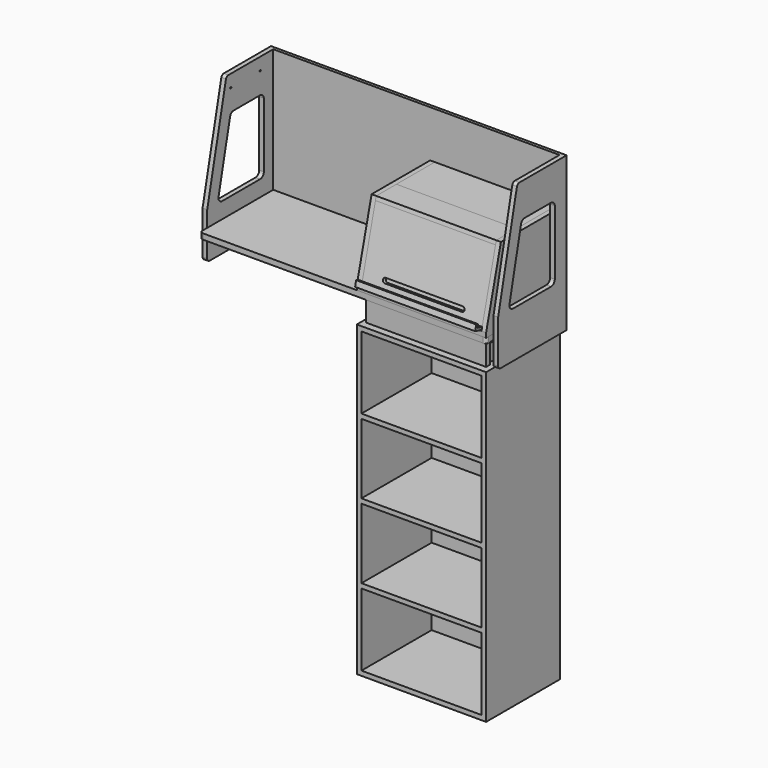
from build123d import *

# Parameters (mm, degrees)
F0_W           = 15
F0_H           = 500
F1_DEPTH       = 8
F2_DEPTH       = 270
F3_SIZE2       = 78
F3_SIZE        = 350
F3_2_SIZE2     = 78
F3_2_SIZE      = 350
F4_W           = 270
F4_H           = 18
F4_W_2         = 30
F5_DEPTH       = 930
F6_R           = 10
F6_2_R         = 10
F7_W           = 15
F7_H           = 235
F7_H_2         = 15
F7_W_2         = 390
F8_DEPTH       = 300
F9_DEPTH       = 8
F10_SIZE2      = 60
F10_SIZE       = 235
F11_W          = 158
F11_H          = 12
F12_DEPTH      = 390
F13_W          = 250
F13_H          = 15
F14_DEPTH      = 25
F15_DEPTH      = 390
F18_DEPTH      = 15
F19_W          = 348
F19_H          = 8
F20_DEPTH      = 285
F19_W_2        = 8
F19_H_2        = 65
F21_DEPTH      = 285
F22_D          = 5
F22_DEPTH      = 12
F22_TIP        = 1.5021515476
F23_DEPTH      = 25
F23_DEPTH_BACK = 945
F24_R          = 15
F26_DEPTH      = 25
F11_W_2        = 150
F11_H_2        = 8
F28_DEPTH      = 390
F27_W          = 152
F27_H          = 8
F29_DEPTH      = 84
F31_DEPTH      = 2
F32_W          = 420
F32_H          = 300
F33_DEPTH      = 1000
F34_T          = -15
F35_W          = 285
F35_H          = 15
F36_DEPTH      = 390


# Not quite as in the source:
# - a feature names something its author has since deleted; it is built from what else it names


with BuildPart() as f1:
    # F0 (on Front) → F1 (new body)
    with BuildSketch(Plane.XZ):
        with Locations((-952.5, 250)):
            Rectangle(F0_W, F0_H)
        with BuildLine():
            Line((-465, 0), (-15, 0))
            Line((-15, 0), (-15, 500))
            Line((-15, 500), (-945, 500))
            Line((-945, 500), (-945, 0))
            Line((-945, 0), (-495, 0))
            ThreePointArc((-495, 0), (-480, 15), (-465, 0))
        make_face()
        with Locations((-7.5, 250)):
            Rectangle(F0_W, F0_H)
    extrude(amount=-F1_DEPTH)

    # F0 (on Front) → F2 (join)
    with BuildSketch(Plane.XZ):
        with Locations((-952.5, 250)):
            Rectangle(F0_W, F0_H)
        with Locations((-7.5, 250)):
            Rectangle(F0_W, F0_H)
    extrude(amount=F2_DEPTH)

    # F3
    f3_edges = [f1.edges().sort_by_distance(p)[0] for p in [
        (-952.5, -270, 500),
    ]]
    f3_side = f1.faces().sort_by_distance((-952.5, -270, 250))[0]
    chamfer(f3_edges, length=F3_SIZE, length2=F3_SIZE2, reference=f3_side)

    # F3#2
    f3_2_edges = [f1.edges().sort_by_distance(p)[0] for p in [
        (-7.5, -270, 500),
    ]]
    f3_2_side = f1.faces().sort_by_distance((-7.5, -270, 250))[0]
    chamfer(f3_2_edges, length=F3_2_SIZE, length2=F3_2_SIZE2, reference=f3_2_side)

    # F6
    f6_edges = [f1.edges().sort_by_distance(p)[0] for p in [
        (-952.5, -192, 500),
        (-7.5, -192, 500),
        (-7.5, -270, 0),
        (-952.5, -270, 0),
    ]]
    fillet(f6_edges, radius=F6_R)

    # F22 (one way)
    with BuildSketch(Plane.YZ.offset(-945)):
        with Locations((-174.4660586119, 460), (-54.8418462276, 460), (-174.4660586119, 80), (-54.8418462276, 80)):
            Circle(F22_D / 2)
    extrude(amount=-F22_DEPTH, mode=Mode.SUBTRACT)
    with Locations(Plane.YZ.offset(-945)):
        with Locations((-174.4660586119, 460), (-54.8418462276, 460), (-174.4660586119, 80), (-54.8418462276, 80)):
            with Locations((0, 0, -(F22_DEPTH + F22_TIP / 2))):  # 118° drill point
                Cone(0, F22_D / 2, F22_TIP, mode=Mode.SUBTRACT)

    # F4 (on face) → F23 (cut, two sides)
    with BuildSketch(Plane.YZ.offset(-945)) as f23_sk:
        Polygon((-40, 390), (-174.4660586119, 390), (-227.9517728976, 150), (-40, 150), align=None)
    extrude(amount=-F23_DEPTH, mode=Mode.SUBTRACT)
    extrude(f23_sk.sketch, amount=F23_DEPTH_BACK, mode=Mode.SUBTRACT)

    # F24
    f24_edges = [f1.edges().sort_by_distance(p)[0] for p in [
        (-952.5, -40, 150),
        (-952.5, -227.951773, 150),
        (-952.5, -40, 390),
        (-7.5, -227.951773, 150),
        (-7.5, -40, 150),
        (-7.5, -40, 390),
        (-7.5, -174.466059, 390),
        (-952.5, -174.466059, 390),
    ]]
    fillet(f24_edges, radius=F24_R)


with BuildPart() as f5:
    # F4 (on face) → F5 (new body, through all)
    with BuildSketch(Plane.YZ.offset(-945)):
        with Locations((-135, 89)):
            Rectangle(F4_W, F4_H)
        with Locations((-285, 89)):
            Rectangle(F4_W_2, F4_H)
    extrude(amount=F5_DEPTH)

    # F6#2
    f6_2_edges = [f5.edges().sort_by_distance(p)[0] for p in [
        (-945, -300, 89),
        (-15, -300, 89),
    ]]
    fillet(f6_2_edges, radius=F6_2_R)

    # F25 (on face) → F26 (cut)
    with BuildSketch(Plane.XY.offset(98)):
        with BuildLine():
            Line((-495, 0), (-465, 0))
            ThreePointArc((-465, 0), (-480, 15), (-495, 0))
        make_face()
        with BuildLine():
            ThreePointArc((-495, 0), (-480, -15), (-465, 0))
            Line((-465, 0), (-495, 0))
        make_face()
    extrude(amount=-F26_DEPTH, mode=Mode.SUBTRACT)


with BuildPart() as f8:
    # F7 (on Front) → F8 (new body)
    with BuildSketch(Plane.XZ):
        with Locations((-427.5, 230.5)):
            Rectangle(F7_W, F7_H)
        with Locations((-427.5, 105.5)):
            Rectangle(F7_W, F7_H_2)
        with Locations((-22.5, 230.5)):
            Rectangle(F7_W, F7_H)
        with Locations((-22.5, 105.5)):
            Rectangle(F7_W, F7_H_2)
        with Locations((-225, 105.5)):
            Rectangle(F7_W_2, F7_H_2)
    extrude(amount=F8_DEPTH)

    # F10
    f10_edges = [f8.edges().sort_by_distance(p)[0] for p in [
        (-427.5, -300, 348),
        (-22.5, -300, 348),
    ]]
    f10_side = f8.faces().sort_by_distance((-427.5, -300, 343.11226))[0]
    chamfer(f10_edges, length=F10_SIZE, length2=F10_SIZE2, reference=f10_side)


with BuildPart() as f9:
    # F7 (on Front) → F9 (new body)
    with BuildSketch(Plane.XZ):
        with Locations((-225, 230.5)):
            Rectangle(F7_W_2, F7_H)
    extrude(amount=F9_DEPTH)

    # F11 (on face) → F28 (join, through all)
    with BuildSketch(Plane.YZ.offset(-420)):
        with Locations((-83, 260)):
            Rectangle(F11_W_2, F11_H_2)
    extrude(amount=F28_DEPTH)

    # F27 (on face) → F29 (join, through all)
    with BuildSketch(Plane.XY.offset(348)):
        Polygon((-182, -8), (-190, -8), (-190, -158), (-182, -158), (-182, -66), (-182, -58), align=None)
        with Locations((-106, -62)):
            Rectangle(F27_W, F27_H)
    extrude(amount=-F29_DEPTH)


with BuildPart() as f12:
    # F11 (on face) → F12 (new body, through all)
    with BuildSketch(Plane.YZ.offset(-420)):
        with Locations((-79, 342)):
            Rectangle(F11_W, F11_H)
        Polygon((-227.6150473168, 348), (-240, 348), (-243.0638297872, 336), (-230.678877104, 336), align=None)
        Polygon((-230.678877104, 336), (-243.0638297872, 336), (-297.2629938822, 123.7199406282), (-299.2420598443, 115.9685989432), (-287.6150473168, 113), align=None)
        Polygon((-299.2420598443, 115.9685989432), (-297.2629938822, 123.7199406282), (-316.1001179345, 128.5294191096), (-313.6262854818, 138.2185962159), (-321.3776271668, 140.197662178), (-325.8305255816, 122.7571433868), align=None)
        Polygon((-158, 348), (-227.6150473168, 348), (-230.678877104, 336), (-158, 336), align=None)
    extrude(amount=F12_DEPTH)

    # F13 (on face) → F14 (cut)
    with BuildSketch(Plane(origin=(0, -308.725881853, 78.8236294093), x_dir=(1, 0, 0), z_dir=(0, -0.9689177106, 0.2473832453))):
        with Locations((-225, 72.618143931)):
            Rectangle(F13_W, F13_H)
        with BuildLine():
            Line((-350, 65.118143931), (-350, 80.118143931))
            ThreePointArc((-350, 80.118143931), (-357.5, 72.618143931), (-350, 65.118143931))
        make_face()
        with BuildLine():
            ThreePointArc((-100, 65.118143931), (-92.5, 72.618143931), (-100, 80.118143931))
            Line((-100, 80.118143931), (-100, 65.118143931))
        make_face()
    extrude(amount=-F14_DEPTH, mode=Mode.SUBTRACT)


with BuildPart() as f15:
    # F11 (on face) → F15 (new body, through all)
    with BuildSketch(Plane.YZ.offset(-420)):
        with Locations((-79, 342)):
            Rectangle(F11_W, F11_H)
    extrude(amount=F15_DEPTH)


with BuildPart() as f12_1:
    add(f12.part)

    # F16: cut F15
    add(f15.part, mode=Mode.SUBTRACT)


with BuildPart() as f18:
    # F17 (on face) → F18 (new body)
    with BuildSketch(Plane.XZ.offset(300)):
        Polygon((-15, 15), (-15, 80), (-25, 80), (-405, 80), (-405, 15), align=None)
    extrude(amount=-F18_DEPTH)


with BuildPart() as f20:
    # F19 (on face) → F20 (new body, through all)
    with BuildSketch(Plane(origin=(0, -285, 0), x_dir=(-1, 0, 0), z_dir=(0, 1, 0))):
        Polygon((24, 68.9618736506), (24, 15), (36, 15), (36, 17.5610594451), (36, 25.5610594451), (36, 68.9618736506), align=None)
        with Locations((210, 21.5610594451)):
            Rectangle(F19_W, F19_H)
        Polygon((384, 17.5610594451), (384, 15), (396, 15), (396, 68.9618736506), (384, 68.9618736506), (384, 25.5610594451), align=None)
    extrude(amount=F20_DEPTH)


with BuildPart() as f21:
    # F19 (on face) → F21 (new body, through all)
    with BuildSketch(Plane(origin=(0, -285, 0), x_dir=(-1, 0, 0), z_dir=(0, 1, 0))):
        with Locations((401, 47.5)):
            Rectangle(F19_W_2, F19_H_2)
    extrude(amount=F21_DEPTH)


with BuildPart() as f31:
    # F30 (on face) → F31 (new body)
    with BuildSketch(Plane.XZ):
        with BuildLine():
            Line((-15, 500), (-945, 500))
            Line((-945, 500), (-945, 0))
            Line((-945, 0), (-495, 0))
            ThreePointArc((-495, 0), (-480, 15), (-465, 0))
            Line((-465, 0), (-15, 0))
            Line((-15, 0), (-15, 500))
        make_face()
    extrude(amount=F31_DEPTH)


with BuildPart() as f33:
    # F32 (on Top) → F33 (new body)
    with BuildSketch(Plane.XY):
        with Locations((-225, -150)):
            Rectangle(F32_W, F32_H)
    extrude(amount=-F33_DEPTH)

    # F34
    f34_openings = [f33.faces().sort_by_distance(p)[0] for p in [
        (-225, -300, -500),
    ]]
    offset(amount=F34_T, openings=f34_openings)

    # F35 (on face) → F36 (join, through all)
    with BuildSketch(Plane.YZ.offset(-420)):
        with Locations((-157.5, -257.5)):
            Rectangle(F35_W, F35_H)
        with Locations((-157.5, -500)):
            Rectangle(F35_W, F35_H)
        with Locations((-157.5, -742.5)):
            Rectangle(F35_W, F35_H)
    extrude(amount=F36_DEPTH)


solid = Compound([f1.part, f5.part, f8.part, f9.part, f15.part, f12_1.part, f18.part, f20.part, f21.part, f31.part, f33.part])
